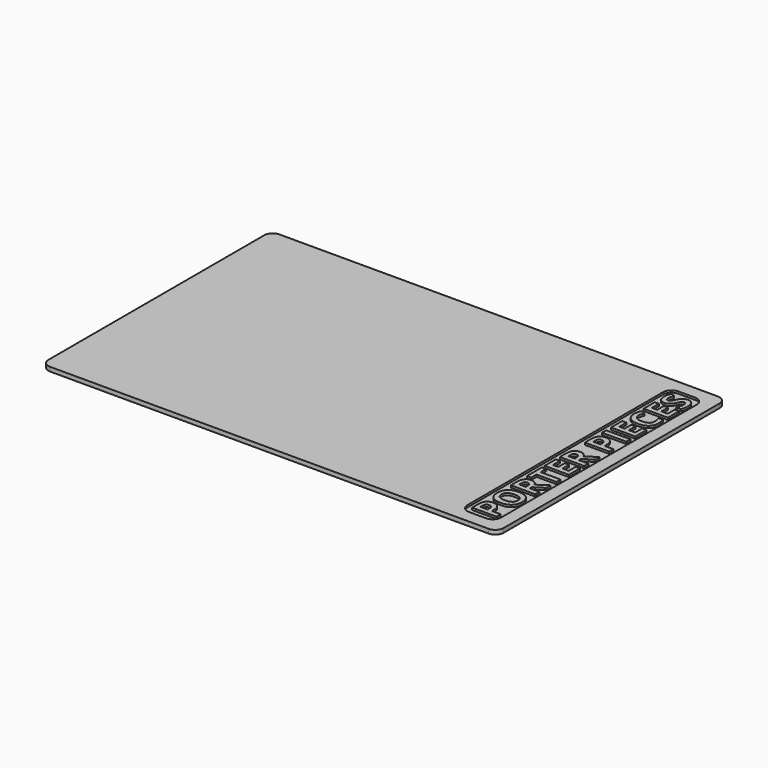
from build123d import *

# Parameters (mm, degrees)
F0_W         = 85.725
F0_H         = 53.975
F1_DEPTH     = 0.79375
F2_R         = 1.5875
F3_W         = 6.35
F3_H         = 49.2125
F4_DEPTH     = 0.396875
F5_R         = 1.5875
F6_TEXT_SIZE = 6.4051106395
F7_DEPTH     = 0.396875


# Not quite as in the source:
# - Text() gives the source's letters only with a copy of the font that has no kerning and outlines rounded to 1/6400 em; it was checked with that copy


with BuildPart() as f1:
    # F0 (on Top) → F1 (new body)
    with BuildSketch(Plane.XY):
        Rectangle(F0_W, F0_H)
    extrude(amount=F1_DEPTH)

    # F2
    f2_edges = [f1.edges().sort_by_distance(p)[0] for p in [
        (42.8625, 26.9875, 0.396875),
        (-42.8625, 26.9875, 0.396875),
        (-42.8625, -26.9875, 0.396875),
        (42.8625, -26.9875, 0.396875),
    ]]
    fillet(f2_edges, radius=F2_R)

    # F3 (on face) → F4 (cut)
    with BuildSketch(Plane.XY.offset(0.79375)):
        with Locations((37.30625, 0)):
            Rectangle(F3_W, F3_H)
    extrude(amount=-F4_DEPTH, mode=Mode.SUBTRACT)

    # F5
    f5_edges = [f1.edges().sort_by_distance(p)[0] for p in [
        (34.13125, -24.60625, 0.595313),
        (40.48125, -24.60625, 0.595313),
        (40.48125, 24.60625, 0.595313),
        (34.13125, 24.60625, 0.595313),
    ]]
    fillet(f5_edges, radius=F5_R)

    # F6 (on face) → F7 (join)
    with BuildSketch(Plane.XY.offset(0.396875)):
        with Locations(Location((39.7566241945, -23.8125), (0, 0, 90))):
            Text('PORTER PIECES', F6_TEXT_SIZE, font='Open Sans', font_style=FontStyle.BOLD, text_align=(TextAlign.LEFT, TextAlign.BOTTOM))
    extrude(amount=F7_DEPTH)


solid = f1.part
